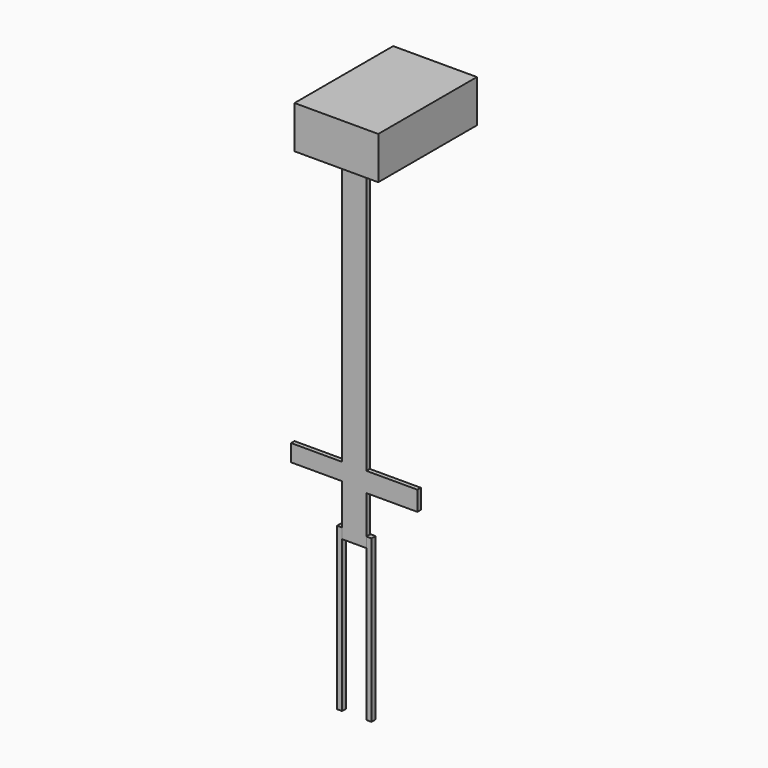
from build123d import *

# Parameters (mm, degrees)
F1_DEPTH  = 950
F2_W      = 142.4321246147
F2_H      = 60
F3_DEPTH  = 25
F4_W      = 142.4321246147
F4_H      = 25
F5_DEPTH  = 340
F6_W      = 25
F6_H      = 115
F7_DEPTH  = 300
F8_W      = 25
F8_H      = 100
F9_DEPTH  = 300
F11_DEPTH = 2000
F12_W     = 142.4321246147
F12_H     = 250
F13_DEPTH = 350
F15_DEPTH = 350
F17_DEPTH = 350


with BuildPart() as f1:
    # F0 (on Top) → F1 (new body)
    with BuildSketch(Plane.XY):
        Polygon((-909.3864560127, -150.3031116724), (-909.3864560127, -160.3031116724), (-909.3864560127, -170.3031116724), (-909.3864560127, -180.3031116724), (-879.3864560127, -180.3031116724), (-879.3864560127, -150.3031116724), align=None)
    extrude(amount=F1_DEPTH)


with BuildPart() as f1b:
    # F0 (on Top) → F1, piece 2 (new body)
    with BuildSketch(Plane.XY):
        Polygon((-1051.8185806274, -150.3031116724), (-1081.8185806274, -150.3031116724), (-1081.8185806274, -180.3031116724), (-1051.8185806274, -180.3031116724), (-1051.8185806274, -170.3031116724), (-1051.8185806274, -165.3031116724), (-1051.8185806274, -160.3031116724), align=None)
    extrude(amount=F1_DEPTH)


with BuildPart() as f3:
    # F2 (on face) → F3 (new body)
    with BuildSketch(Plane.XZ.offset(180.3031116724)):
        with Locations((-980.6025183201, 920)):
            Rectangle(F2_W, F2_H)
    extrude(amount=-F3_DEPTH)

    # F4 (on face) → F5 (join)
    with BuildSketch(Plane.XY.offset(950)):
        with Locations((-980.6025183201, -167.8031116724)):
            Rectangle(F4_W, F4_H)
    extrude(amount=F5_DEPTH)

    # F6 (on face) → F7 (join)
    with BuildSketch(Plane.YZ.offset(-909.3864560127)):
        with Locations((-167.8031116724, 1232.5)):
            Rectangle(F6_W, F6_H)
    extrude(amount=F7_DEPTH)

    # F8 (on face) → F9 (join)
    with BuildSketch(Plane(origin=(-1051.8185806274, 0, 0), x_dir=(0, -1, 0), z_dir=(-1, 0, 0))):
        with Locations((167.8031116724, 1240)):
            Rectangle(F8_W, F8_H)
    extrude(amount=F9_DEPTH)

    # F10 (on face) → F11 (join)
    with BuildSketch(Plane.XY.offset(1290)):
        Polygon((-1051.8185806274, -180.3031116724), (-909.3864560127, -180.3031116724), (-1051.8185806274, -155.3031116724), align=None)
        Polygon((-1051.8185806274, -155.3031116724), (-909.3864560127, -180.3031116724), (-909.3864560127, -155.3031116724), align=None)
    extrude(amount=F11_DEPTH)

    # F12 (on face) → F13 (join)
    with BuildSketch(Plane.XZ.offset(180.3031116724)):
        with Locations((-980.6025183201, 3165)):
            Rectangle(F12_W, F12_H)
    extrude(amount=F13_DEPTH)

    # F14 (on face) → F15 (join)
    with BuildSketch(Plane.YZ.offset(-909.3864560127)):
        Polygon((-530.3031116724, 3040), (-180.3031116724, 3040), (-155.3031116724, 3040), (-155.3031116724, 3290), (-530.3031116724, 3290), align=None)
    extrude(amount=F15_DEPTH)

    # F16 (on face) → F17 (join)
    with BuildSketch(Plane(origin=(0, -155.3031116724, 0), x_dir=(-1, 0, 0), z_dir=(0, 1, 0))):
        Polygon((559.3864560127, 3040), (909.3864560127, 3040), (1051.8185806274, 3040), (1051.8185806274, 3290), (559.3864560127, 3290), align=None)
    extrude(amount=F17_DEPTH)


solid = Compound([f1.part, f1b.part, f3.part])
